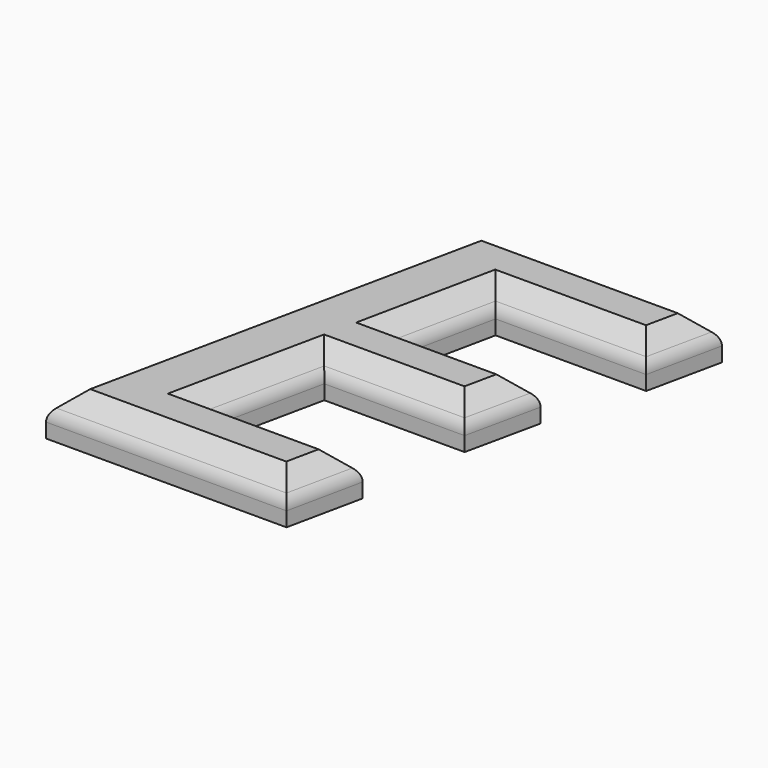
from build123d import *

# Parameters (mm, degrees)
F0_TEXT_SIZE = 176.3888888889
F1_DEPTH     = 12.7
F2_SIZE      = 6.35
F3_R         = 5.08


# Not quite as in the source:
# - Text() gives the source's letters only with a copy of the font that has no kerning and outlines rounded to 1/6400 em; it was checked with that copy


with BuildPart() as f1:
    # F0 (on Top) → F1 (new body)
    with BuildSketch(Plane.XY):
        with Locations((-56.5604207107, -64.6874927639)):
            Text('E', F0_TEXT_SIZE, font='Open Sans', font_style=FontStyle.BOLDITALIC, text_align=(TextAlign.LEFT, TextAlign.BOTTOM))
    extrude(amount=F1_DEPTH)

    # F2
    f2_edges = [f1.edges().sort_by_distance(p)[0] for p in [
        (-16.804019, -64.687493, 12.7),
        (20.706181, -53.663187, 12.7),
        (0.986454, -42.638882, 12.7),
        (-17.617061, -26.405592, 12.7),
        (6.360803, -10.172302, 12.7),
        (29.263798, 0.769321, 12.7),
        (11.087474, 11.710945, 12.7),
        (-6.565195, 25.532668, 12.7),
        (18.377296, 39.354391, 12.7),
        (42.754792, 50.296014, 12.7),
        (9.84724, 61.237637, 12.7),
        (-38.687265, -1.724928, 12.7),
    ]]
    chamfer(f2_edges, length=F2_SIZE)

    # F3
    f3_edges = [f1.edges().sort_by_distance(p)[0] for p in [
        (9.84724, 61.237637, 6.35),
        (-38.687265, -1.724928, 6.35),
        (42.754792, 50.296014, 6.35),
        (18.377296, 39.354391, 6.35),
        (-6.565195, 25.532668, 6.35),
        (11.087474, 11.710945, 6.35),
        (29.263798, 0.769321, 6.35),
        (6.360803, -10.172302, 6.35),
        (-17.617061, -26.405592, 6.35),
        (0.986454, -42.638882, 6.35),
        (20.706181, -53.663187, 6.35),
        (-16.804019, -64.687493, 6.35),
    ]]
    fillet(f3_edges, radius=F3_R)


solid = f1.part
